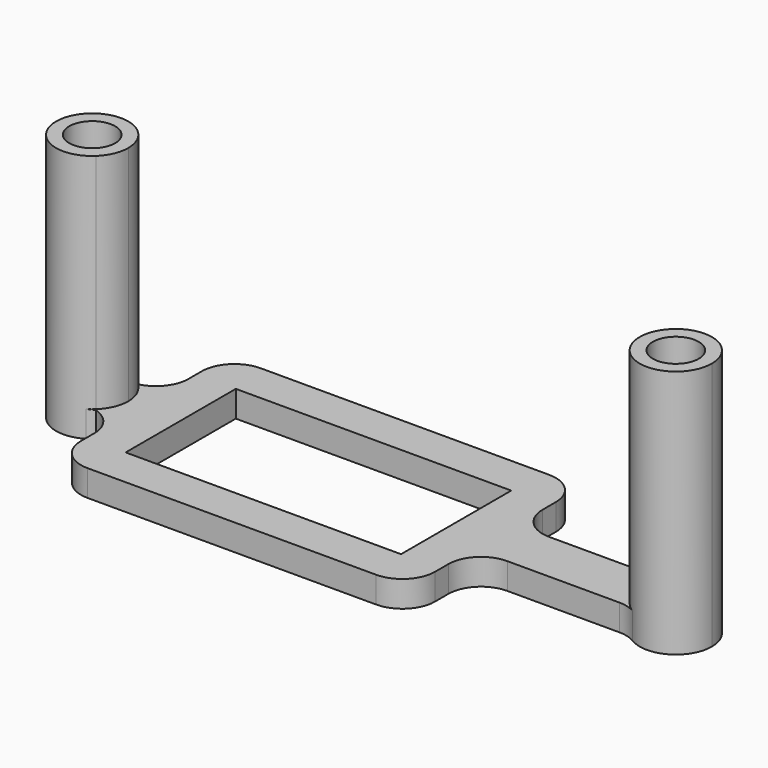
from build123d import *

# Parameters (mm, degrees)
F1_DEPTH    = 4
F0_R        = 3.5
F2_DEPTH    = 38
F0_W        = 6
F0_H        = 8
F3_DEPTH    = 4
F4_T1_DEPTH = 4
F4_T3_DEPTH = 29


# Not quite as in the source:
# - a fillet or chamfer that OpenCascade refuses, or shapes differently, is made with other operations: its cross-section is extruded or revolved along the edge and cut away or added


with BuildPart() as f1:
    # F0 (on Top) → F1 (new body)
    with BuildSketch(Plane.XY):
        with BuildLine():
            ThreePointArc((-40.7250827824, 4), (-39.4496512647, 2.1780674121), (-39, 0))
            ThreePointArc((-39, 0), (-39.4496512647, -2.1780674121), (-40.7250827824, -4))
            Line((-40.7250827824, -4), (-37, -4))
            Line((-37, -4), (-37, 4))
            Line((-37, 4), (-40.7250827824, 4))
        make_face()
    extrude(amount=F1_DEPTH)

    # F0 (on Top) → F2 (join)
    with BuildSketch(Plane.XY):
        with BuildLine():
            ThreePointArc((-40.7250827824, -4), (-39.4496512647, -2.1780674121), (-39, 0))
            ThreePointArc((-39, 0), (-39.4496512647, 2.1780674121), (-40.7250827824, 4))
            ThreePointArc((-40.7250827824, 4), (-50, 0), (-40.7250827824, -4))
        make_face()
        with Locations((-44.5, 0)):
            Circle(F0_R, mode=Mode.SUBTRACT)
    extrude(amount=F2_DEPTH)



with BuildPart() as f1b:
    # F0 (on Top) → F1, piece 2 (new body)
    with BuildSketch(Plane.XY):
        with BuildLine():
            Line((40.7250827824, 4), (17, 4))
            Line((17, 4), (17, -4))
            Line((17, -4), (40.7250827824, -4))
            ThreePointArc((40.7250827824, -4), (39, 0), (40.7250827824, 4))
        make_face()
    extrude(amount=F1_DEPTH)

    # F0 (on Top) → F2, piece 2 (join)
    with BuildSketch(Plane.XY):
        with BuildLine():
            ThreePointArc((50, 0), (46.6780674121, 5.0503487353), (40.7250827824, 4))
            ThreePointArc((40.7250827824, 4), (39, 0), (40.7250827824, -4))
            ThreePointArc((40.7250827824, -4), (46.6780674121, -5.0503487353), (50, 0))
        make_face()
        with Locations((44.5, 0)):
            Circle(F0_R, mode=Mode.SUBTRACT)
    extrude(amount=F2_DEPTH)


with BuildPart() as f1_1:
    add(f1.part)

    add(f1b.part)  # F3 merges F1b
    # F0 (on Top) → F3 (join)
    with BuildSketch(Plane.XY):
        Polygon((-31, -4), (-37, -4), (-37, -16.5), (17, -16.5), (17, -4), (11, -4), (11, -10.5), (-31, -10.5), align=None)
        Polygon((-37, 16.5), (-37, 4), (-31, 4), (-31, 10.5), (11, 10.5), (11, 4), (17, 4), (17, 16.5), align=None)
        with Locations((-34, 0)):
            Rectangle(F0_W, F0_H)
        with Locations((14, 0)):
            Rectangle(F0_W, F0_H)
    extrude(amount=F3_DEPTH)

    # F4: fillet of radius 5 on 12 edges, made by hand

    # F4_s2 → F4_t1 (join)
    with BuildSketch(Plane.XY):
        with BuildLine():
            ThreePointArc((-39.0916730868, 4), (-40.4279792964, 4.1818794417), (-41.667066855, 4.7142857143))
            ThreePointArc((-41.667066855, 4.7142857143), (-41.1768279274, 4.3825252282), (-40.7250827824, 4))
            Line((-40.7250827824, 4), (-39.0916730868, 4))
        make_face()
        with BuildLine():
            ThreePointArc((-37, 9), (-38.4644660941, 5.4644660941), (-42, 4))
            Line((-42, 4), (-37, 4))
            Line((-37, 4), (-37, 9))
        make_face()
        with BuildLine():
            ThreePointArc((-37, -9), (-38.4644660941, -5.4644660941), (-42, -4))
            Line((-42, -4), (-37, -4))
            Line((-37, -4), (-37, -9))
        make_face()
        with BuildLine():
            ThreePointArc((-39.0916730868, -4), (-40.4279792964, -4.1818794417), (-41.667066855, -4.7142857143))
            ThreePointArc((-41.667066855, -4.7142857143), (-41.1768279274, -4.3825252282), (-40.7250827824, -4))
            Line((-40.7250827824, -4), (-39.0916730868, -4))
        make_face()
        with BuildLine():
            ThreePointArc((17, 9), (18.4644660941, 5.4644660941), (22, 4))
            Line((22, 4), (17, 4))
            Line((17, 4), (17, 9))
        make_face()
        with BuildLine():
            ThreePointArc((17, -9), (18.4644660941, -5.4644660941), (22, -4))
            Line((22, -4), (17, -4))
            Line((17, -4), (17, -9))
        make_face()
        with BuildLine():
            ThreePointArc((39.0916730868, -4), (40.4279792964, -4.1818794417), (41.667066855, -4.7142857143))
            ThreePointArc((41.667066855, -4.7142857143), (41.1768279274, -4.3825252282), (40.7250827824, -4))
            Line((40.7250827824, -4), (39.0916730868, -4))
        make_face()
        with BuildLine():
            ThreePointArc((41.667066855, 4.7142857143), (40.4279792964, 4.1818794417), (39.0916730868, 4))
            Line((39.0916730868, 4), (40.7250827824, 4))
            ThreePointArc((40.7250827824, 4), (41.1768279274, 4.3825252282), (41.667066855, 4.7142857143))
        make_face()
    extrude(amount=F4_T1_DEPTH)

    # F4_s4 → F4_t3 (cut)
    with BuildSketch(Plane.XY.offset(-12.5)):
        with BuildLine():
            ThreePointArc((12, 16.5), (15.5355339059, 15.0355339059), (17, 11.5))
            Line((17, 11.5), (17, 16.5))
            Line((17, 16.5), (12, 16.5))
        make_face()
        with BuildLine():
            ThreePointArc((-37, 11.5), (-35.5355339059, 15.0355339059), (-32, 16.5))
            Line((-32, 16.5), (-37, 16.5))
            Line((-37, 16.5), (-37, 11.5))
        make_face()
        with BuildLine():
            ThreePointArc((-32, -16.5), (-35.5355339059, -15.0355339059), (-37, -11.5))
            Line((-37, -11.5), (-37, -16.5))
            Line((-37, -16.5), (-32, -16.5))
        make_face()
        with BuildLine():
            ThreePointArc((12, -16.5), (15.5355339059, -15.0355339059), (17, -11.5))
            Line((17, -11.5), (17, -16.5))
            Line((17, -16.5), (12, -16.5))
        make_face()
    extrude(amount=F4_T3_DEPTH, mode=Mode.SUBTRACT)


solid = f1_1.part
